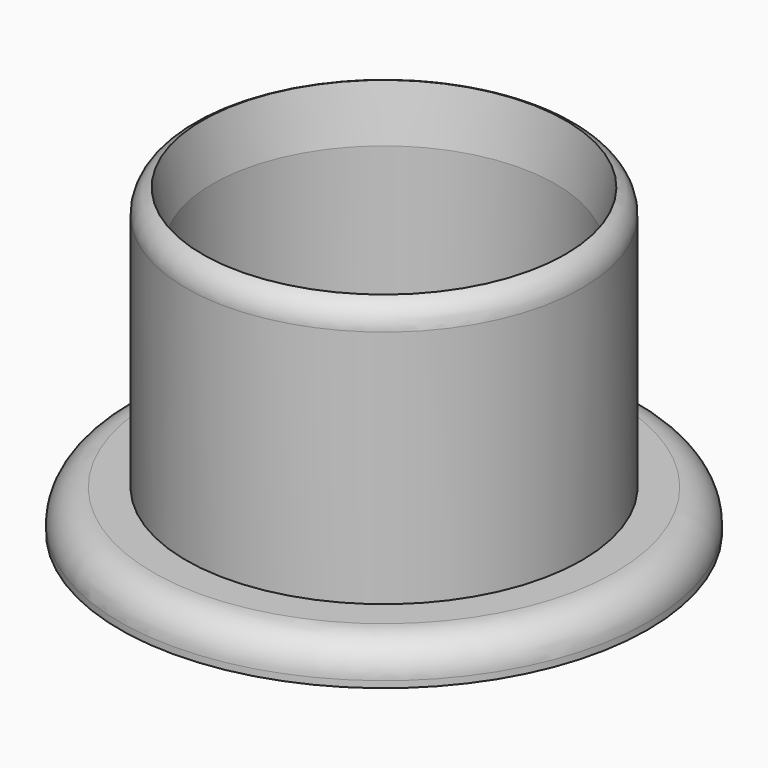
from build123d import *

# Parameters (mm, degrees)
F0_R     = 20
F0_R_2   = 13
F1_DEPTH = 3
F2_R     = 15
F2_R_2   = 13
F3_DEPTH = 20
F4_R     = 2.5
F5_SIZE2 = 4
F5_SIZE  = 0.75


# Not quite as in the source:
# - a fillet or chamfer that OpenCascade refuses, or shapes differently, is made with other operations: its cross-section is extruded or revolved along the edge and cut away or added


with BuildPart() as f1:
    # F0 (on Top) → F1 (new body)
    with BuildSketch(Plane.XY):
        Circle(F0_R)
        Circle(F0_R_2, mode=Mode.SUBTRACT)
    extrude(amount=F1_DEPTH)

    # F2 (on face) → F3 (join)
    with BuildSketch(Plane.XY.offset(3)):
        Circle(F2_R)
        Circle(F2_R_2, mode=Mode.SUBTRACT)
    extrude(amount=F3_DEPTH)

    # F4
    f4_edges = [f1.edges().sort_by_distance(p)[0] for p in [
        (-20, 0, 3),
    ]]
    fillet(f4_edges, radius=F4_R)

    # F5
    f5_edges = [f1.edges().sort_by_distance(p)[0] for p in [
        (-13, 0, 23),
    ]]
    f5_side = f1.faces().sort_by_distance((-14.575736, 0, 23))[0]
    chamfer(f5_edges, length=F5_SIZE, length2=F5_SIZE2, reference=f5_side)

    # F6: fillet of radius 2 on 1 edges, made by hand

    # F6_s1 → F6_t2 (revolve, cut)
    with BuildSketch(Plane.XZ):
        with BuildLine():
            ThreePointArc((13.75, 23), (14.6583123952, 22.263984367), (15, 21.1459503782))
            Line((15, 21.1459503782), (15, 23))
            Line((15, 23), (13.75, 23))
        make_face()
    revolve(axis=Axis((0, 0, 23), (0, 0, 1)), mode=Mode.SUBTRACT)


solid = f1.part
